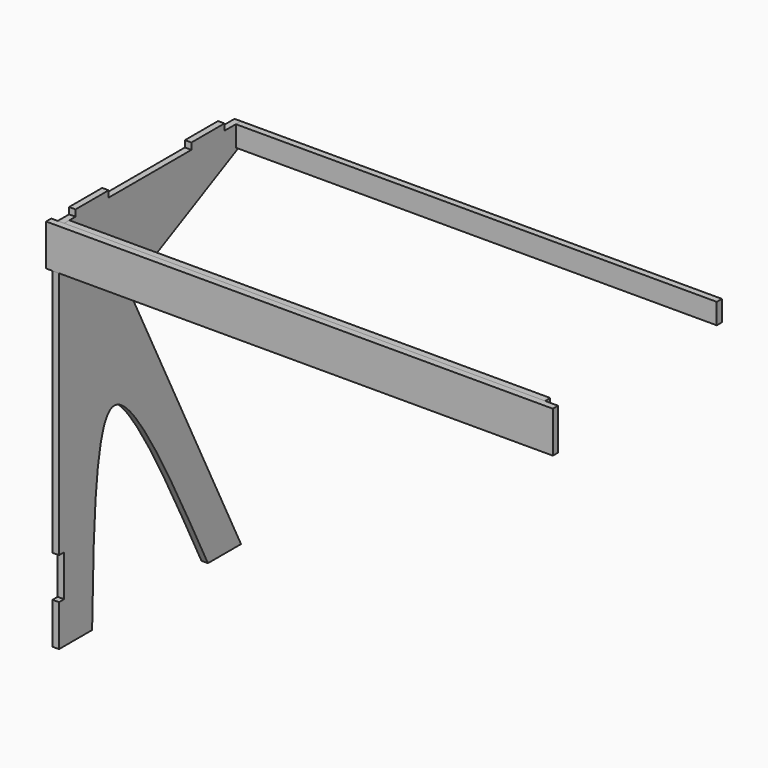
from build123d import *

# Parameters (mm, degrees)
F1_DEPTH      = 15.875
F2_W          = 15.875
F2_H          = 50.8
F3_DEPTH      = 1181.1
F4_W          = 15.875
F4_H          = 101.6
F5_DEPTH      = 1181.1
F6_W          = 15.875
F6_H          = 101.6
F7_DEPTH      = 1212.85
F7_DEPTH_BACK = 31.75


with BuildPart() as f1:
    # F0 (on Right) → F1 (new body)
    with BuildSketch(Plane.YZ):
        with BuildLine():
            Line((-492.125, 489.6790781498), (-508, 489.6790781498))
            Line((-508, 489.6790781498), (-508, -119.9209218502))
            Line((-508, -119.9209218502), (-492.125, -119.9209218502))
            Line((-492.125, -119.9209218502), (-492.125, -221.5209218502))
            Line((-492.125, -221.5209218502), (-508, -221.5209218502))
            Line((-508, -221.5209218502), (-508, -323.1209218502))
            Line((-508, -323.1209218502), (-406.4, -323.1209218502))
            add(Edge.make_bspline(
                [(-406.4, -323.1209218502), (-401.7010466691, -100.4355481062), (-391.907715593, 363.674528608), (-167.5225646264, -88.1085703651), (-50.8, -323.1209218502)],
                knots=[0, 0, 0, 0, 0.4798115467, 1, 1, 1, 1], degree=3))
            Line((-50.8, -323.1209218502), (50.8, -323.1209218502))
            Line((50.8, -323.1209218502), (-294.64, 367.7590781498))
            Line((-294.64, 367.7590781498), (50.8, 540.4790781498))
            Line((50.8, 540.4790781498), (50.8, 591.2790781498))
            Line((50.8, 591.2790781498), (0, 591.2790781498))
            Line((0, 591.2790781498), (0, 607.1540781498))
            Line((0, 607.1540781498), (-101.6, 607.1540781498))
            Line((-101.6, 607.1540781498), (-101.6, 591.2790781498))
            Line((-101.6, 591.2790781498), (-355.6, 591.2790781498))
            Line((-355.6, 591.2790781498), (-355.6, 607.1540781498))
            Line((-355.6, 607.1540781498), (-457.2, 607.1540781498))
            Line((-457.2, 607.1540781498), (-457.2, 591.2790781498))
            Line((-457.2, 591.2790781498), (-492.125, 591.2790781498))
            Line((-492.125, 591.2790781498), (-492.125, 489.6790781498))
        make_face()
    extrude(amount=F1_DEPTH)


with BuildPart() as f3:
    # F2 (on face) → F3 (new body)
    with BuildSketch(Plane.YZ.offset(15.875)):
        with Locations((42.8625, 565.8790781498)):
            Rectangle(F2_W, F2_H)
    extrude(amount=F3_DEPTH)


with BuildPart() as f5:
    # F4 (on face) → F5 (new body)
    with BuildSketch(Plane.YZ.offset(15.875)):
        with Locations((-484.1875, 540.4790781498)):
            Rectangle(F4_W, F4_H)
    extrude(amount=F5_DEPTH)


with BuildPart() as f7:
    # F6 (on face) → F7 (new body, two sides)
    with BuildSketch(Plane.YZ.offset(15.875)) as f7_sk:
        with Locations((-500.0625, 540.4790781498)):
            Rectangle(F6_W, F6_H)
    extrude(amount=F7_DEPTH)
    extrude(f7_sk.sketch, amount=-F7_DEPTH_BACK)


solid = Compound([f1.part, f3.part, f5.part, f7.part])
